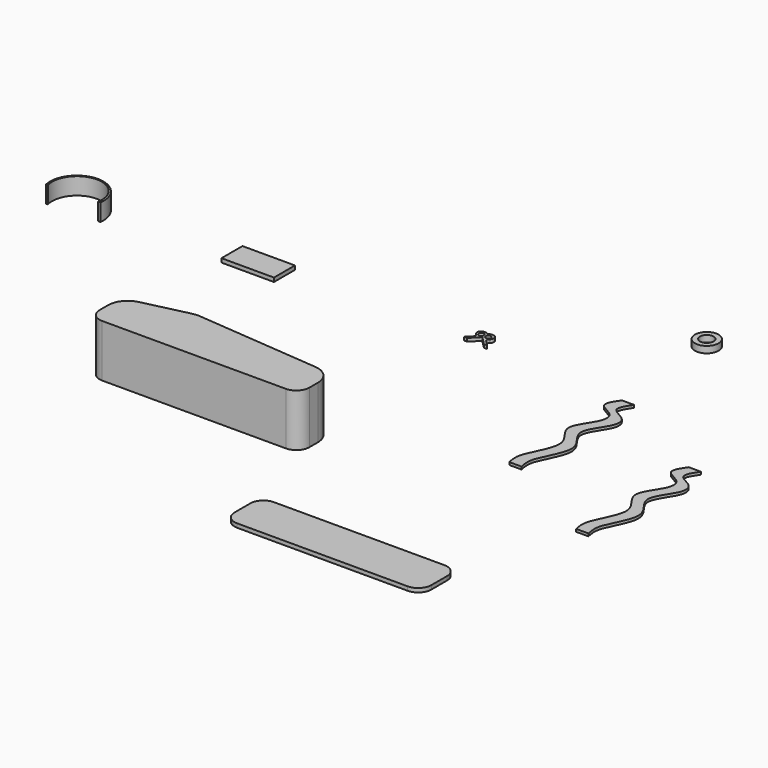
from build123d import *

# Parameters (mm, degrees)
F1_DEPTH  = 10.16
F3_DEPTH  = 8.382
F4_W      = 6.8476469303
F4_H      = 9.144
F5_DEPTH  = 5.08
F6_R      = 0.5007069219
F7_DEPTH  = 0.635
F9_DEPTH  = 3.302
F11_DEPTH = 0.508
F12_DEPTH = 0.508
F14_DEPTH = 0.762
F15_R     = 2.2924687411
F15_R_2   = 1.3171780173
F16_DEPTH = 1.27
F17_W     = 10.16
F17_H     = 5.08
F18_DEPTH = 0.762


# Not quite as in the source:
# - ends of sketch curves that miss each other by under 0.0002 mm in the source are joined


with BuildPart() as f1:
    # F0 (on Top) → F1 (new body)
    with BuildSketch(Plane.XY):
        with BuildLine():
            ThreePointArc((-24.7868363938, 8.3085960276), (-26.9037898481, 6.9661045557), (-27.7284322733, 4.5988825234))
            Line((-27.7284322733, 4.5988825234), (-27.7284322733, 2.54))
            ThreePointArc((-27.7284322733, 2.54), (-26.9844834975, 0.7439487758), (-25.1884322733, 0))
            Line((-25.1884322733, 0), (10.3715677267, 0))
            ThreePointArc((10.3715677267, 0), (12.1676189509, 0.7439487758), (12.9115677267, 2.54))
            Line((12.9115677267, 2.54), (12.9115677267, 4.5988825234))
            ThreePointArc((12.9115677267, 4.5988825234), (11.9081590401, 7.1755364), (9.4264521363, 8.3950055615))
            Line((9.4264521363, 8.3950055615), (-14.5522111368, 10.4471766271))
            ThreePointArc((-14.5522111368, 10.4471766271), (-15.345923724, 10.4528693603), (-16.1308346038, 10.3348566959))
            Line((-16.1308346038, 10.3348566959), (-16.1432625103, 10.3319639152))
            Line((-16.1432625103, 10.3319639152), (-24.7868363938, 8.3085960276))
        make_face()
    extrude(amount=F1_DEPTH)

    # F2 (on face) → F3 (cut)
    with BuildSketch(Plane(origin=(0.7817892721, 9.1348435917, 0), x_dir=(-0.9963577528, 0.0852714986, 0), z_dir=(0.0852714986, 0.9963577528, 0))):
        with BuildLine():
            Line((15.3900547932, 0.508), (15.3900547932, 9.652))
            Line((15.3900547932, 9.652), (-5.253791913, 9.652))
            ThreePointArc((-5.253791913, 9.652), (-7.2709161912, 9.0742298257), (-8.6762639624, 7.5161520454))
            Line((-8.6762639624, 7.5161520454), (-8.6762639624, 2.6438479546))
            ThreePointArc((-8.6762639624, 2.6438479546), (-7.2709161912, 1.0857701743), (-5.253791913, 0.508))
            Line((-5.253791913, 0.508), (15.3900547932, 0.508))
        make_face()
    extrude(amount=-F3_DEPTH, mode=Mode.SUBTRACT)

    # F4 (on face) → F5 (cut)
    with BuildSketch(Plane(origin=(-15.334000409, 1.3123330354, 0), x_dir=(0.0852714986, 0.9963577528, 0), z_dir=(0.9963577528, -0.0852714986, 0))):
        with Locations((4.2100600409, 5.08)):
            Rectangle(F4_W, F4_H)
    extrude(amount=-F5_DEPTH, mode=Mode.SUBTRACT)


with BuildPart() as f7:
    # F6 (on Top) → F7 (new body)
    with BuildSketch(Plane.XY):
        with BuildLine():
            Line((10.332825936, 45.4332928986), (9.3346098438, 44.4234013557))
            Line((9.3346098438, 44.4234013557), (9.9642197122, 44.4234013557))
            Line((9.9642197122, 44.4234013557), (11.5771517158, 46.0551987213))
            Line((11.5771517158, 46.0551987213), (13.1900837193, 44.4234013557))
            Line((13.1900837193, 44.4234013557), (13.8196935877, 44.4234013557))
            Line((13.8196935877, 44.4234013557), (12.8214774955, 45.4332928986))
            ThreePointArc((12.8214774955, 45.4332928986), (12.6751603345, 45.8103155683), (12.850554154, 46.1747216785))
            Line((12.850554154, 46.1747216785), (12.9423046835, 46.2540345991))
            ThreePointArc((12.9423046835, 46.2540345991), (13.1945501477, 46.9619938139), (12.7166629365, 47.5420436715))
            ThreePointArc((12.7166629365, 47.5420436715), (12.4932857662, 47.6049423658), (12.2621925548, 47.6261445728))
            ThreePointArc((12.2621925548, 47.6261445728), (11.8948137983, 47.5573978913), (11.5771517158, 47.3604612052))
            ThreePointArc((11.5771517158, 47.3604612052), (11.2594896332, 47.5573978913), (10.8921108767, 47.6261445728))
            ThreePointArc((10.8921108767, 47.6261445728), (10.6610176653, 47.6049423658), (10.4376404951, 47.5420436715))
            ThreePointArc((10.4376404951, 47.5420436715), (9.9597532838, 46.9619938139), (10.211998748, 46.2540345991))
            Line((10.211998748, 46.2540345991), (10.3037492775, 46.1747216785))
            ThreePointArc((10.3037492775, 46.1747216785), (10.4791430971, 45.8103155683), (10.332825936, 45.4332928986))
        make_face()
        with Locations((10.8921108767, 46.6637188027)):
            Circle(F6_R, mode=Mode.SUBTRACT)
        with Locations((12.2621925548, 46.6637188027)):
            Circle(F6_R, mode=Mode.SUBTRACT)
    extrude(amount=F7_DEPTH)


with BuildPart() as f9:
    # F8 (on Top) → F9 (new body)
    with BuildSketch(Plane.XY):
        with BuildLine():
            Line((-58.2907013595, 40.3810308359), (-57.8335013595, 40.3810308359))
            ThreePointArc((-57.8335013595, 40.3810308359), (-63.1833058582, 46.2103688914), (-67.9935013595, 39.9283620799))
            Line((-67.9935013595, 39.9283620799), (-67.6338970661, 39.9283620799))
            ThreePointArc((-67.6338970661, 39.9283620799), (-63.2441257914, 45.9716671324), (-58.2907013595, 40.3810308359))
        make_face()
    extrude(amount=F9_DEPTH)


with BuildPart() as f11:
    # F10 (on Top) → F11 (new body)
    with BuildSketch(Plane.XY):
        with BuildLine():
            Line((43.196901679, 43.2678200305), (40.8197306097, 43.2678200305))
            add(Edge.make_bspline(
                [(40.8197306097, 43.2678200305), (40.0903424352, 42.1875066472), (38.6401764766, 40.0396329251), (42.7687162109, 38.9513613115), (42.8981542778, 35.6961252098), (38.3864305973, 30.863637368), (44.2964114797, 26.8628834056), (39.4633863407, 20.0726945137), (39.9567922733, 17.775361978), (40.1539243758, 16.8575011194)],
                knots=[0, 0, 0, 0, 0.1248190868, 0.2481646906, 0.3642220301, 0.5286341512, 0.6867855887, 0.8748604114, 1, 1, 1, 1], degree=3))
            Line((40.1539243758, 16.8575011194), (42.5310954452, 16.8575011194))
            add(Edge.make_bspline(
                [(43.196901679, 43.2678200305), (42.4675135046, 42.1875066472), (41.017347546, 40.0396329251), (45.1458872803, 38.9513613115), (45.2753253472, 35.6961252098), (40.7636016667, 30.863637368), (46.6735825491, 26.8628834056), (41.8405574101, 20.0726945137), (42.3339633426, 17.775361978), (42.5310954452, 16.8575011194)],
                knots=[0, 0, 0, 0, 0.1248190868, 0.2481646906, 0.3642220301, 0.5286341512, 0.6867855887, 0.8748604114, 1, 1, 1, 1], degree=3))
        make_face()
    extrude(amount=F11_DEPTH)

    # F10 (on Top) → F12 (join)
    with BuildSketch(Plane.XY):
        with BuildLine():
            Line((43.196901679, 43.2678200305), (40.8197306097, 43.2678200305))
            add(Edge.make_bspline(
                [(40.8197306097, 43.2678200305), (40.0903424352, 42.1875066472), (38.6401764766, 40.0396329251), (42.7687162109, 38.9513613115), (42.8981542778, 35.6961252098), (38.3864305973, 30.863637368), (44.2964114797, 26.8628834056), (39.4633863407, 20.0726945137), (39.9567922733, 17.775361978), (40.1539243758, 16.8575011194)],
                knots=[0, 0, 0, 0, 0.1248190868, 0.2481646906, 0.3642220301, 0.5286341512, 0.6867855887, 0.8748604114, 1, 1, 1, 1], degree=3))
            Line((40.1539243758, 16.8575011194), (42.5310954452, 16.8575011194))
            add(Edge.make_bspline(
                [(43.196901679, 43.2678200305), (42.4675135046, 42.1875066472), (41.017347546, 40.0396329251), (45.1458872803, 38.9513613115), (45.2753253472, 35.6961252098), (40.7636016667, 30.863637368), (46.6735825491, 26.8628834056), (41.8405574101, 20.0726945137), (42.3339633426, 17.775361978), (42.5310954452, 16.8575011194)],
                knots=[0, 0, 0, 0, 0.1248190868, 0.2481646906, 0.3642220301, 0.5286341512, 0.6867855887, 0.8748604114, 1, 1, 1, 1], degree=3))
        make_face()
    extrude(amount=F12_DEPTH)


with BuildPart() as f12:
    # F10 (on Top) → F12, piece 2 (new body)
    with BuildSketch(Plane.XY):
        with BuildLine():
            Line((64.7716616045, 32.4967515558), (62.3944905351, 32.4967515558))
            add(Edge.make_bspline(
                [(62.3944905351, 32.4967515558), (61.6651023607, 31.4164381725), (60.2149364021, 29.2685644504), (64.3434761363, 28.1802928369), (64.4729142032, 24.9250567351), (59.9611905228, 20.0925688934), (65.8711714052, 16.091814931), (61.0381462662, 9.301626039), (61.5315521987, 7.0042935034), (61.7286843012, 6.0864326447)],
                knots=[0, 0, 0, 0, 0.1248190868, 0.2481646906, 0.3642220301, 0.5286341512, 0.6867855887, 0.8748604114, 1, 1, 1, 1], degree=3))
            Line((61.7286843012, 6.0864326447), (64.1058553706, 6.0864326447))
            add(Edge.make_bspline(
                [(64.7716616045, 32.4967515558), (64.0422734301, 31.4164381725), (62.5921074715, 29.2685644504), (66.7206472057, 28.1802928369), (66.8500852726, 24.9250567351), (62.3383615921, 20.0925688934), (68.2483424746, 16.091814931), (63.4153173355, 9.301626039), (63.9087232681, 7.0042935034), (64.1058553706, 6.0864326447)],
                knots=[0, 0, 0, 0, 0.1248190868, 0.2481646906, 0.3642220301, 0.5286341512, 0.6867855887, 0.8748604114, 1, 1, 1, 1], degree=3))
        make_face()
    extrude(amount=F12_DEPTH)


with BuildPart() as f14:
    # F13 (on Top) → F14 (new body)
    with BuildSketch(Plane.XY):
        with BuildLine():
            Line((53.89424927, -16.0089726677), (20.87424927, -16.0089726677))
            ThreePointArc((20.87424927, -16.0089726677), (19.0781980457, -16.7529214435), (18.33424927, -18.5489726677))
            Line((18.33424927, -18.5489726677), (18.33424927, -22.3589726677))
            ThreePointArc((18.33424927, -22.3589726677), (19.0781980457, -24.1550238919), (20.87424927, -24.8989726677))
            Line((20.87424927, -24.8989726677), (53.89424927, -24.8989726677))
            ThreePointArc((53.89424927, -24.8989726677), (55.6903004942, -24.1550238919), (56.43424927, -22.3589726677))
            Line((56.43424927, -22.3589726677), (56.43424927, -18.5489726677))
            ThreePointArc((56.43424927, -18.5489726677), (55.6903004942, -16.7529214435), (53.89424927, -16.0089726677))
        make_face()
    extrude(amount=F14_DEPTH)


with BuildPart() as f16:
    # F15 (on Top) → F16 (new body)
    with BuildSketch(Plane.XY):
        with Locations((39.2073839903, 65.8483356237)):
            Circle(F15_R)
        with Locations((39.2073839903, 65.8483356237)):
            Circle(F15_R_2, mode=Mode.SUBTRACT)
    extrude(amount=F16_DEPTH)


with BuildPart() as f18:
    # F17 (on Top) → F18 (new body)
    with BuildSketch(Plane.XY):
        with Locations((-30.1450286061, 43.965123704)):
            Rectangle(F17_W, F17_H)
    extrude(amount=F18_DEPTH)


solid = Compound([f1.part, f7.part, f9.part, f11.part, f12.part, f14.part, f16.part, f18.part])
